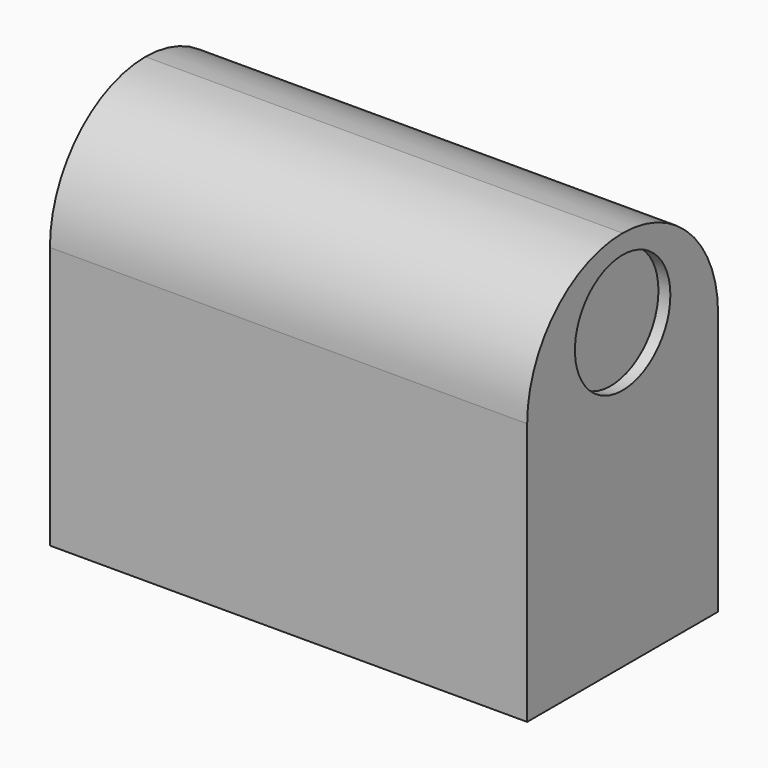
from build123d import *

# Parameters (mm, degrees)
F0_W     = 500
F0_H     = 800
F1_DEPTH = 1000
F2_R     = 125
F3_DEPTH = 25
F4_R     = 249.99999
F6_DEPTH = 25
F7_W     = 600
F7_H     = 8.0311238766
F8_DEPTH = 100


# Not quite as in the source:
# - a fillet or chamfer is up to 0.001 mm smaller than in the source, because OpenCascade refuses the exact size


with BuildPart() as f1:
    # F0 (on Right) → F1 (new body)
    with BuildSketch(Plane.YZ):
        Rectangle(F0_W, F0_H)
    extrude(amount=F1_DEPTH)

    # F2 (on face) → F3 (cut)
    with BuildSketch(Plane.YZ.offset(1000)):
        with Locations((0, 234.9280565977)):
            Circle(F2_R)
    extrude(amount=-F3_DEPTH, mode=Mode.SUBTRACT)

    # F4 (radius 250 in the source; OpenCascade refuses exactly that, so slightly less here)
    f4_edges = [f1.edges().sort_by_distance(p)[0] for p in [
        (500, 250, 400),
        (500, -250, 400),
    ]]
    fillet(f4_edges, radius=F4_R)

    # F5 (on face) → F6 (cut)
    with BuildSketch(Plane(origin=(0, 250, 0), x_dir=(-1, 0, 0), z_dir=(0, 1, 0))):
        Polygon((-300, 150), (-700, 150), (-700, -14.3443720028), (-700, -150), (-300, -150), align=None)
    extrude(amount=-F6_DEPTH, mode=Mode.SUBTRACT)

    # F7 (on face) → F8 (cut)
    with BuildSketch(Plane(origin=(0, 250, 0), x_dir=(-1, 0, 0), z_dir=(0, 1, 0))):
        with Locations((-500, -404.0155619383)):
            Rectangle(F7_W, F7_H)
    extrude(amount=-F8_DEPTH, mode=Mode.SUBTRACT)


solid = f1.part
